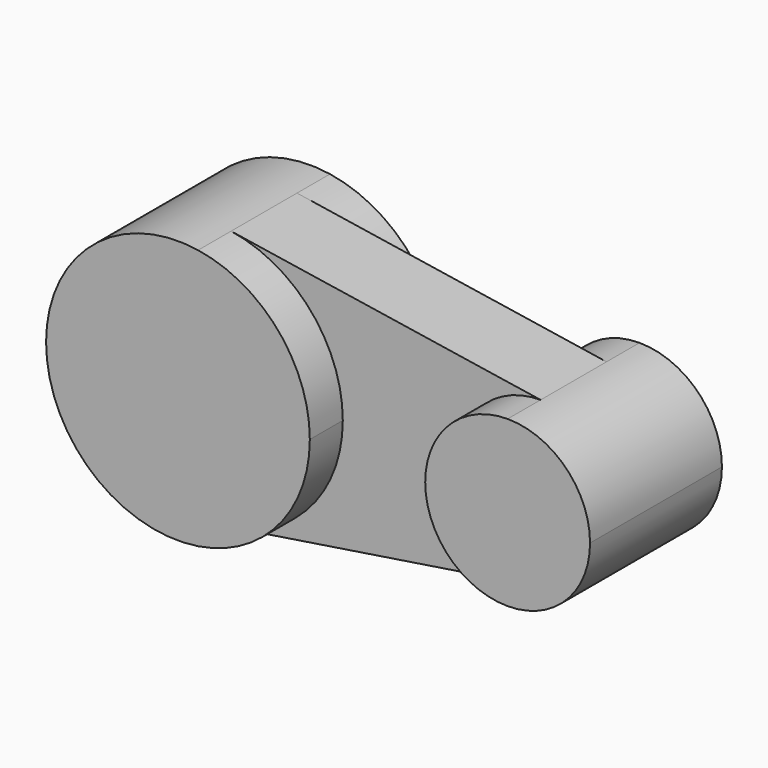
from build123d import *

# Parameters (mm, degrees)
F1_DEPTH = 6.35
F2_DEPTH = 6.35
F3_DEPTH = 3.175


with BuildPart() as f1:
    # F0 (on Front) → F1 (new body, symmetric)
    with BuildSketch(Plane.XZ):
        with BuildLine():
            ThreePointArc((1.553882, -10.040471), (7.714047, -6.61204), (10.16, 0))
            ThreePointArc((10.16, 0), (7.714047, 6.61204), (1.553882, 10.040471))
            ThreePointArc((1.553882, 10.040471), (-10.16, 0), (1.553882, -10.040471))
        make_face()
    extrude(amount=F1_DEPTH, both=True)


with BuildPart() as f2:
    # F0 (on Front) → F2 (new body, symmetric)
    with BuildSketch(Plane.XZ):
        with BuildLine():
            ThreePointArc((25.4, 6.35), (20.909872, 4.490128), (19.05, 0))
            ThreePointArc((19.05, 0), (20.909872, -4.490128), (25.4, -6.35))
            ThreePointArc((25.4, -6.35), (29.890128, -4.490128), (31.75, 0))
            ThreePointArc((31.75, 0), (29.890128, 4.490128), (25.4, 6.35))
        make_face()
    extrude(amount=F2_DEPTH, both=True)


with BuildPart() as f3:
    # F0 (on Front) → F3 (new body, symmetric)
    with BuildSketch(Plane.XZ):
        with BuildLine():
            ThreePointArc((1.553882, 10.040471), (7.714047, 6.61204), (10.16, 0))
            Line((10.16, 0), (19.05, 0))
            ThreePointArc((19.05, 0), (20.909872, 4.490128), (25.4, 6.35))
            Line((25.4, 6.35), (1.553882, 10.040471))
        make_face()
        with BuildLine():
            Line((19.05, 0), (10.16, 0))
            ThreePointArc((10.16, 0), (7.714047, -6.61204), (1.553882, -10.040471))
            Line((1.553882, -10.040471), (25.4, -6.35))
            ThreePointArc((25.4, -6.35), (20.909872, -4.490128), (19.05, 0))
        make_face()
    extrude(amount=F3_DEPTH, both=True)


solid = Compound([f1.part, f2.part, f3.part])
